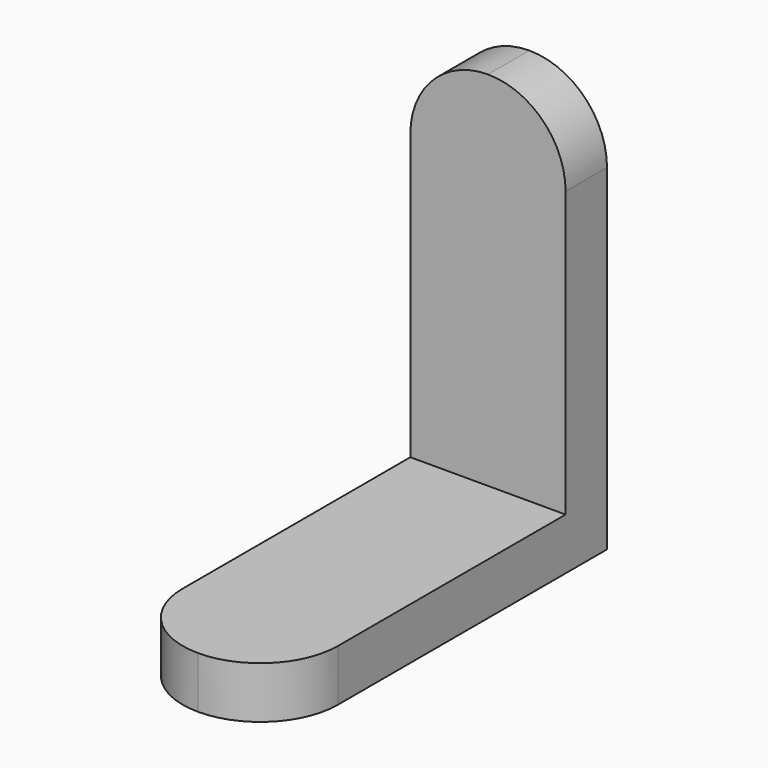
from build123d import *

# Parameters (mm, degrees)
F1_DEPTH = 9.525
F2_R     = 9.52499


# Not quite as in the source:
# - a fillet or chamfer is up to 0.001 mm smaller than in the source, because OpenCascade refuses the exact size


with BuildPart() as f1:
    # F0 (on Right) → F1 (new body, symmetric)
    with BuildSketch(Plane.YZ):
        Polygon((-50.8, 6.35), (-50.8, 0), (0, 0), (0, 50.8), (-6.35, 50.8), (-6.35, 6.35), align=None)
    extrude(amount=F1_DEPTH, both=True)

    # F2 (radius 9.525 in the source; OpenCascade refuses exactly that, so slightly less here)
    f2_edges = [f1.edges().sort_by_distance(p)[0] for p in [
        (9.525, -3.175, 50.8),
        (-9.525, -3.175, 50.8),
        (9.525, -50.8, 3.175),
        (-9.525, -50.8, 3.175),
    ]]
    fillet(f2_edges, radius=F2_R)


solid = f1.part
